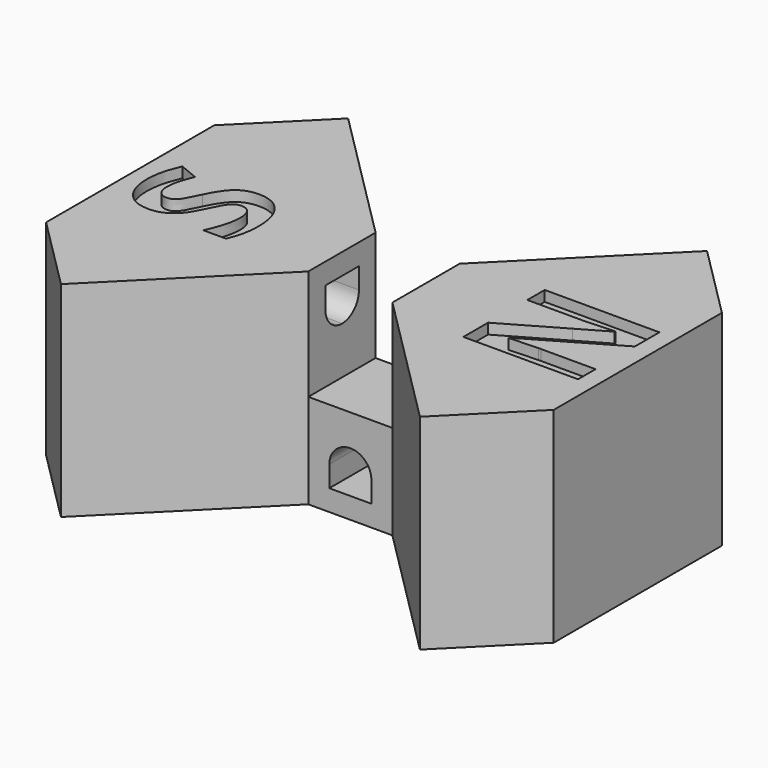
from build123d import *

# Parameters (mm, degrees)
F1_DEPTH      = 19.5
F2_DEPTH      = 9
F3_W          = 2
F3_H          = 2
F4_DEPTH      = 8
F5_W          = 2
F5_H          = 2
F6_DEPTH      = 15
F7_W          = 2
F7_H          = 2
F8_DEPTH      = 15
F10_DEPTH     = 1
F11_TEXT_SIZE = 15.2777777778
F12_DEPTH     = 1
F13_TEXT_SIZE = 15.2777777778
F14_DEPTH     = 1
F15_TEXT_SIZE = 15.2777777778
F16_DEPTH     = 1


# Not quite as in the source:
# - Text() gives the source's letters only with a copy of the font that has no kerning and outlines rounded to 1/6400 em; it was checked with that copy


with BuildPart() as f1:
    # F0 (on Top) → F1 (new body)
    with BuildSketch(Plane.XY):
        Polygon((-17.0710678119, 17.0710678119), (-24.1421356237, 10), (-24.1421356237, -10), (-17.0710678119, -17.0710678119), (-4, -4), (-4, 4), align=None)
    extrude(amount=F1_DEPTH)



with BuildPart() as f1b:
    # F0 (on Top) → F1, piece 2 (new body)
    with BuildSketch(Plane.XY):
        Polygon((17.0710678119, 17.0710678119), (4, 4), (4, -4), (17.0710678119, -17.0710678119), (24.1421356237, -10), (24.1421356237, 10), align=None)
    extrude(amount=F1_DEPTH)


with BuildPart() as f1_1:
    add(f1.part)

    add(f1b.part)  # F2 merges F1b
    # F0 (on Top) → F2 (join)
    with BuildSketch(Plane.XY):
        Polygon((4, 4), (0, 0), (4, -4), align=None)
        Polygon((4, 4), (-4, 4), (0, 0), align=None)
        Polygon((0, 0), (-4, 4), (-4, -4), align=None)
        Polygon((4, -4), (0, 0), (-4, -4), align=None)
    extrude(amount=F2_DEPTH)

    # F3 (on face) → F4 (cut)
    with BuildSketch(Plane.XZ.offset(4)):
        with Locations((1, 3)):
            Rectangle(F3_W, F3_H)
        with Locations((-1, 3)):
            Rectangle(F3_W, F3_H)
        with BuildLine():
            ThreePointArc((0, 6), (-1.4142135624, 5.4142135624), (-2, 4))
            Line((-2, 4), (0, 4))
            Line((0, 4), (0, 6))
        make_face()
        with BuildLine():
            Line((0, 6), (0, 4))
            Line((0, 4), (2, 4))
            ThreePointArc((2, 4), (1.4142135624, 5.4142135624), (0, 6))
        make_face()
    extrude(amount=-F4_DEPTH, mode=Mode.SUBTRACT)

    # F5 (on face) → F6 (cut)
    with BuildSketch(Plane.YZ.offset(-4)):
        with Locations((-0.976299841, 16.5)):
            Rectangle(F5_W, F5_H)
        with Locations((1.023700159, 16.5)):
            Rectangle(F5_W, F5_H)
        with BuildLine():
            Line((0.023700159, 13.5), (0.023700159, 15.5))
            Line((0.023700159, 15.5), (-1.976299841, 15.5))
            ThreePointArc((-1.976299841, 15.5), (-1.3905134033, 14.0857864376), (0.023700159, 13.5))
        make_face()
        with BuildLine():
            ThreePointArc((0.023700159, 13.5), (1.4379137214, 14.0857864376), (2.023700159, 15.5))
            Line((2.023700159, 15.5), (0.023700159, 15.5))
            Line((0.023700159, 15.5), (0.023700159, 13.5))
        make_face()
    extrude(amount=-F6_DEPTH, mode=Mode.SUBTRACT)

    # F7 (on face) → F8 (cut)
    with BuildSketch(Plane(origin=(4, 0, 0), x_dir=(0, -1, 0), z_dir=(-1, 0, 0))):
        with Locations((1, 16.5)):
            Rectangle(F7_W, F7_H)
        with Locations((-1, 16.5)):
            Rectangle(F7_W, F7_H)
        with BuildLine():
            ThreePointArc((-2, 15.5), (0, 13.5), (2, 15.5))
            Line((2, 15.5), (0, 15.5))
            Line((0, 15.5), (-2, 15.5))
        make_face()
    extrude(amount=-F8_DEPTH, mode=Mode.SUBTRACT)

    # F9 (on face) → F10 (cut)
    with BuildSketch(Plane.XY.offset(19.5)):
        with BuildLine():
            Line((17.0710678119, 2.5837623701), (17.0710678119, 4.6465928819))
            Line((17.0710678119, 4.6465928819), (11.5710678119, 4.6465928819))
            Line((11.5710678119, 4.6465928819), (11.5710678119, 2.5793185764))
            Line((11.5710678119, 2.5793185764), (16.7034462841, 2.5793185764))
            add(Edge.make_bspline(
                [(17.0710678119, 2.5837623701), (16.867852482, 2.5793185764), (16.7034462841, 2.5793185764)],
                knots=[0.8238586933, 0.8238586933, 0.8238586933, 1, 1, 1], degree=2))
        make_face()
        with BuildLine():
            Line((22.4779688535, 4.6465928819), (17.0710678119, 4.6465928819))
            Line((17.0710678119, 4.6465928819), (17.0710678119, 2.5837623701))
            add(Edge.make_bspline(
                [(19.8210678119, 2.7225477431), (18.0215587519, 2.604547149), (17.0710678119, 2.5837623701)],
                knots=[0, 0, 0, 0.8238586933, 0.8238586933, 0.8238586933], degree=2))
            Line((19.8210678119, 2.7225477431), (19.8210678119, 2.6557074653))
            Line((19.8210678119, 2.6557074653), (17.0710678119, 1.0738208912))
            Line((17.0710678119, 1.0738208912), (17.0710678119, -1.4053095853))
            Line((17.0710678119, -1.4053095853), (22.4779688535, 1.7294921875))
            Line((22.4779688535, 1.7294921875), (22.4779688535, 4.6465928819))
        make_face()
        with BuildLine():
            Line((17.0710678119, -1.4053095853), (17.0710678119, 1.0738208912))
            Line((17.0710678119, 1.0738208912), (11.5710678119, -2.0899522569))
            Line((11.5710678119, -2.0899522569), (11.5710678119, -5.0285373264))
            Line((11.5710678119, -5.0285373264), (17.0710678119, -5.0285373264))
            Line((17.0710678119, -5.0285373264), (17.0710678119, -2.9487527525))
            add(Edge.make_bspline(
                [(14.309132048, -3.0591362847), (16.1657356169, -2.9612009674), (17.0710678119, -2.9487527525)],
                knots=[0, 0, 0, 0.8728935053, 0.8728935053, 0.8728935053], degree=2))
            Line((14.309132048, -3.0591362847), (14.309132048, -3.0066189236))
            Line((14.309132048, -3.0066189236), (17.0710678119, -1.4053095853))
        make_face()
        with BuildLine():
            Line((17.0710678119, -2.9487527525), (17.0710678119, -5.0285373264))
            Line((17.0710678119, -5.0285373264), (22.4779688535, -5.0285373264))
            Line((22.4779688535, -5.0285373264), (22.4779688535, -2.9469401042))
            Line((22.4779688535, -2.9469401042), (17.3145573952, -2.9469401042))
            add(Edge.make_bspline(
                [(17.0710678119, -2.9487527525), (17.2028978703, -2.9469401042), (17.3145573952, -2.9469401042)],
                knots=[0.8728935053, 0.8728935053, 0.8728935053, 1, 1, 1], degree=2))
        make_face()
    extrude(amount=-F10_DEPTH, mode=Mode.SUBTRACT)

    # F11 (on face) → F12 (cut)
    with BuildSketch(Plane.XY.offset(19.5)):
        with Locations(Location((-11.5710678119, -4.4007161458), (0, 0, 90))):
            Text('S', F11_TEXT_SIZE, font='Open Sans', font_style=FontStyle.BOLD, text_align=(TextAlign.LEFT, TextAlign.BOTTOM))
    extrude(amount=-F12_DEPTH, mode=Mode.SUBTRACT)

    # F13 (on face) → F14 (cut)
    with BuildSketch(Plane.XY):
        with Locations(Location((11.5710678119, 7.8811848958), (0, 0, -90))):
            Text('W', F13_TEXT_SIZE, font='Open Sans', font_style=FontStyle.BOLD, text_align=(TextAlign.LEFT, TextAlign.BOTTOM))
    extrude(amount=F14_DEPTH, mode=Mode.SUBTRACT)

    # F15 (on face) → F16 (cut)
    with BuildSketch(Plane.XY):
        with Locations(Location((-22.5710678119, 4.3219401042), (0, 0, -90))):
            Text('E', F15_TEXT_SIZE, font='Open Sans', font_style=FontStyle.BOLD, text_align=(TextAlign.LEFT, TextAlign.BOTTOM))
    extrude(amount=F16_DEPTH, mode=Mode.SUBTRACT)


solid = f1_1.part
